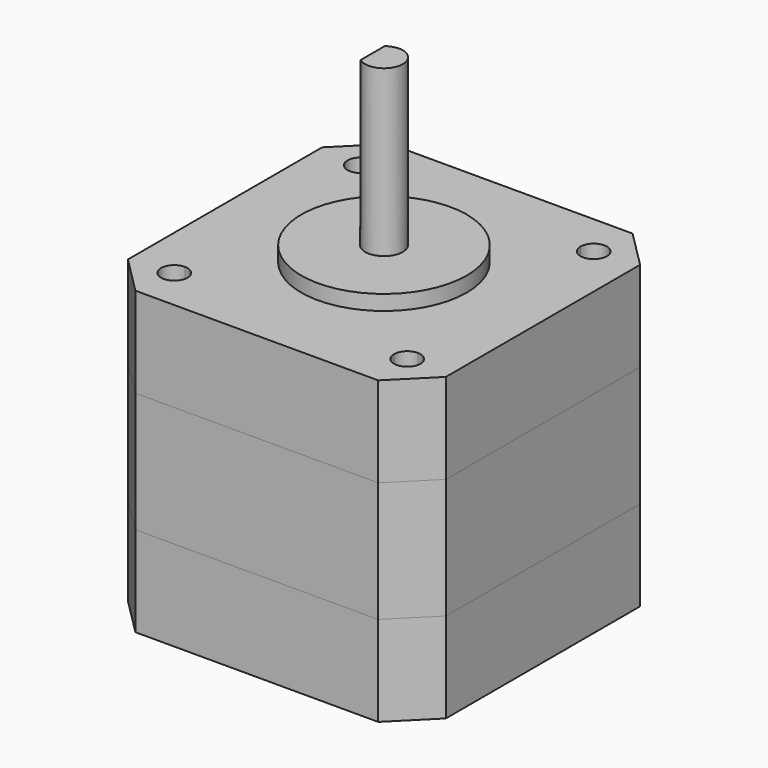
from build123d import *

# Parameters (mm, degrees)
F0_W      = 42.3
F0_H      = 42.3
F1_DEPTH  = 12
F2_SIZE   = 5
F3_W      = 42.3
F3_H      = 42.3
F4_DEPTH  = 16
F5_SIZE   = 5
F6_W      = 42.3
F6_H      = 42.3
F7_DEPTH  = 12
F8_SIZE   = 5
F9_R      = 11
F10_DEPTH = 12
F11_R     = 11
F11_R_2   = 2.5
F12_DEPTH = 14
F13_R     = 2.5
F14_DEPTH = 36
F16_DEPTH = 20


with BuildPart() as f1:
    # F0 (on Top) → F1 (new body)
    with BuildSketch(Plane.XY):
        Rectangle(F0_W, F0_H)
    extrude(amount=F1_DEPTH)

    # F2
    f2_edges = [f1.edges().sort_by_distance(p)[0] for p in [
        (21.15, -21.15, 6),
        (21.15, 21.15, 6),
        (-21.15, -21.15, 6),
        (-21.15, 21.15, 6),
    ]]
    chamfer(f2_edges, length=F2_SIZE)


with BuildPart() as f4:
    # F3 (on face) → F4 (new body)
    with BuildSketch(Plane.XY.offset(12)):
        Rectangle(F3_W, F3_H)
    extrude(amount=F4_DEPTH)

    # F5
    f5_edges = [f4.edges().sort_by_distance(p)[0] for p in [
        (21.15, -21.15, 20),
        (21.15, 21.15, 20),
        (-21.15, -21.15, 20),
        (-21.15, 21.15, 20),
    ]]
    chamfer(f5_edges, length=F5_SIZE)


with BuildPart() as f7:
    # F6 (on face) → F7 (new body)
    with BuildSketch(Plane.XY.offset(28)):
        Rectangle(F6_W, F6_H)
    extrude(amount=F7_DEPTH)

    # F8
    f8_edges = [f7.edges().sort_by_distance(p)[0] for p in [
        (21.15, -21.15, 34),
        (21.15, 21.15, 34),
        (-21.15, 21.15, 34),
        (-21.15, -21.15, 34),
    ]]
    chamfer(f8_edges, length=F8_SIZE)

    # F9 (on face) → F10 (cut)
    with BuildSketch(Plane.XY.offset(40)):
        with BuildLine():
            Line((15.5, 15.5), (13.75, 15.5))
            ThreePointArc((13.75, 15.5), (14.2625631329, 14.2625631329), (15.5, 13.75))
            Line((15.5, 13.75), (15.5, 15.5))
        make_face()
        with BuildLine():
            ThreePointArc((17.25, 15.5), (15.5, 17.25), (13.75, 15.5))
            Line((13.75, 15.5), (15.5, 15.5))
            Line((15.5, 15.5), (15.5, 13.75))
            ThreePointArc((15.5, 13.75), (16.7374368671, 14.2625631329), (17.25, 15.5))
        make_face()
        with BuildLine():
            ThreePointArc((-15.5, 13.75), (-14.2625631329, 14.2625631329), (-13.75, 15.5))
            Line((-13.75, 15.5), (-15.5, 15.5))
            Line((-15.5, 15.5), (-15.5, 13.75))
        make_face()
        with BuildLine():
            Line((-15.5, 15.5), (-13.75, 15.5))
            ThreePointArc((-13.75, 15.5), (-16.7374368671, 16.7374368671), (-15.5, 13.75))
            Line((-15.5, 13.75), (-15.5, 15.5))
        make_face()
        with BuildLine():
            Line((15.5, -15.5), (15.5, -13.75))
            ThreePointArc((15.5, -13.75), (14.2625631329, -14.2625631329), (13.75, -15.5))
            Line((13.75, -15.5), (15.5, -15.5))
        make_face()
        with BuildLine():
            ThreePointArc((17.25, -15.5), (16.7374368671, -14.2625631329), (15.5, -13.75))
            Line((15.5, -13.75), (15.5, -15.5))
            Line((15.5, -15.5), (13.75, -15.5))
            ThreePointArc((13.75, -15.5), (15.5, -17.25), (17.25, -15.5))
        make_face()
        with BuildLine():
            ThreePointArc((-13.75, -15.5), (-14.2625631329, -14.2625631329), (-15.5, -13.75))
            Line((-15.5, -13.75), (-15.5, -15.5))
            Line((-15.5, -15.5), (-13.75, -15.5))
        make_face()
        with BuildLine():
            Line((-15.5, -15.5), (-15.5, -13.75))
            ThreePointArc((-15.5, -13.75), (-16.7374368671, -16.7374368671), (-13.75, -15.5))
            Line((-13.75, -15.5), (-15.5, -15.5))
        make_face()
        Circle(F9_R)
    extrude(amount=-F10_DEPTH, mode=Mode.SUBTRACT)


with BuildPart() as f12:
    # F11 (on face) → F12 (new body)
    with BuildSketch(Plane.XY.offset(28)):
        Circle(F11_R)
        Circle(F11_R_2, mode=Mode.SUBTRACT)
    extrude(amount=F12_DEPTH)


with BuildPart() as f14:
    # F13 (on face) → F14 (new body)
    with BuildSketch(Plane.XY.offset(28)):
        Circle(F13_R)
    extrude(amount=F14_DEPTH)

    # F15 (on face) → F16 (cut)
    with BuildSketch(Plane.XY.offset(64)):
        with BuildLine():
            Line((-1.5, -2), (-1.5, 0))
            Line((-1.5, 0), (-1.5, 2))
            ThreePointArc((-1.5, 2), (-2.5, 0), (-1.5, -2))
        make_face()
    extrude(amount=-F16_DEPTH, mode=Mode.SUBTRACT)


solid = Compound([f1.part, f4.part, f7.part, f12.part, f14.part])
